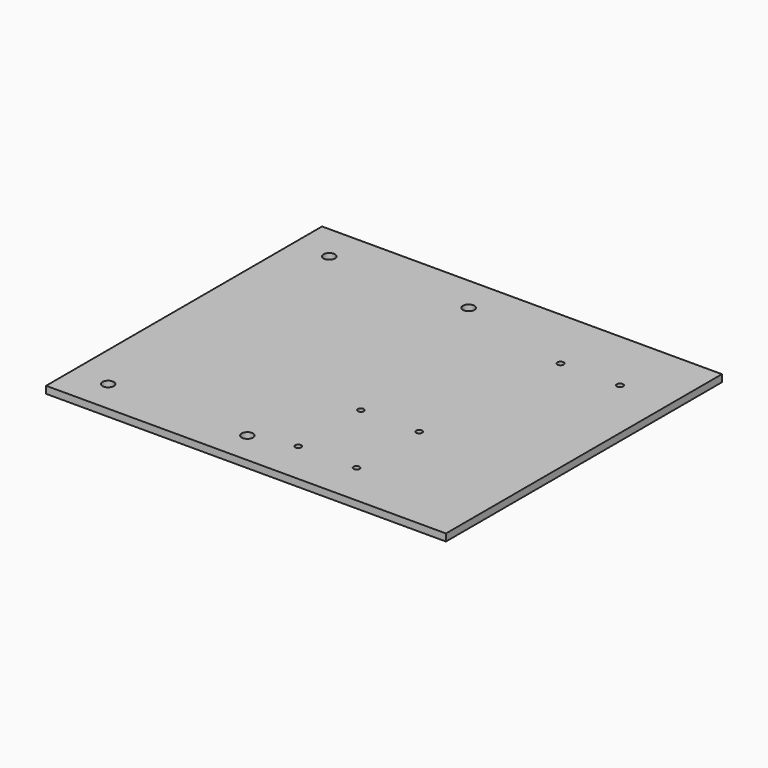
from build123d import *

# Parameters (mm, degrees)
F0_W     = 26
F0_H     = 35.5
F0_W_2   = 45
F0_H_2   = 10
F0_R     = 2
F0_R_2   = 1.05
F0_W_3   = 15
F0_R_3   = 1.1
F1_DEPTH = 2.5


with BuildPart() as f1:
    # F0 (on Top) → F1 (new body)
    with BuildSketch(Plane.XY):
        Polygon((-81.5970200658, 98.7071764616), (-96.5970200658, 98.7071764616), (-96.5970200658, -22.0728235384), (43.4029799342, -22.0728235384), (43.4029799342, 98.7071764616), (-36.5970200658, 98.7071764616), (-36.5970200658, 88.7071764616), (-35.1970200658, 88.7071764616), (-32.5970200658, 88.7071764616), (-32.5970200658, 86.1071764616), (-32.5970200658, -10.6928235384), (-32.5970200658, -13.2928235384), (-35.1970200658, -13.2928235384), (-83.9970200658, -13.2928235384), (-86.5970200658, -13.2928235384), (-86.5970200658, -10.6928235384), (-86.5970200658, 86.1071764616), (-86.5970200658, 86.5071764616), (-86.5970200658, 88.7071764616), (-84.3970200658, 88.7071764616), (-83.9970200658, 88.7071764616), (-81.5970200658, 88.7071764616), align=None)
        Polygon((-23.1610157355, -9.7928235384), (-23.1610157355, 23.2071764616), (-17.1610157355, 23.2071764616), (-17.1610157355, 33.2071764616), (-2.1610157355, 33.2071764616), (-2.1610157355, 23.2071764616), (2.8389842645, 23.2071764616), (2.8389842645, -9.7928235384), align=None, mode=Mode.SUBTRACT)
        with Locations((15.4029799342, 60.9571764616)):
            Rectangle(F0_W, F0_H, mode=Mode.SUBTRACT)
        with Locations((-59.0970200658, 93.7071764616)):
            Rectangle(F0_W_2, F0_H_2)
        Polygon((-36.5970200658, 88.7071764616), (-81.5970200658, 88.7071764616), (-83.9970200658, 88.7071764616), (-84.3970200658, 88.7071764616), (-86.5970200658, 88.7071764616), (-86.5970200658, 86.5071764616), (-86.5970200658, 86.1071764616), (-86.5970200658, -10.6928235384), (-86.5970200658, -13.2928235384), (-83.9970200658, -13.2928235384), (-35.1970200658, -13.2928235384), (-32.5970200658, -13.2928235384), (-32.5970200658, -10.6928235384), (-32.5970200658, 86.1071764616), (-32.5970200658, 88.7071764616), (-35.1970200658, 88.7071764616), align=None)
        with Locations((-83.9970200658, -10.6928235384)):
            Circle(F0_R, mode=Mode.SUBTRACT)
        with Locations((-35.1970200658, -10.6928235384)):
            Circle(F0_R, mode=Mode.SUBTRACT)
        with Locations((-83.9970200658, 86.1071764616)):
            Circle(F0_R, mode=Mode.SUBTRACT)
        with Locations((-35.1970200658, 86.1071764616)):
            Circle(F0_R, mode=Mode.SUBTRACT)
        Polygon((-17.1610157355, 23.2071764616), (-23.1610157355, 23.2071764616), (-23.1610157355, -9.7928235384), (2.8389842645, -9.7928235384), (2.8389842645, 23.2071764616), (-2.1610157355, 23.2071764616), align=None)
        with Locations((-20.3610157355, -6.9928235384)):
            Circle(F0_R_2, mode=Mode.SUBTRACT)
        with Locations((0.0389842645, -6.9928235384)):
            Circle(F0_R_2, mode=Mode.SUBTRACT)
        with Locations((-20.3610157355, 20.4071764616)):
            Circle(F0_R_2, mode=Mode.SUBTRACT)
        with Locations((0.0389842645, 20.4071764616)):
            Circle(F0_R_2, mode=Mode.SUBTRACT)
        with Locations((-9.6610157355, 28.2071764616)):
            Rectangle(F0_W_3, F0_H_2)
        with Locations((15.4029799342, 60.9571764616)):
            Rectangle(F0_W, F0_H)
        with Locations((5.0029799342, 76.1071764616)):
            Circle(F0_R_3, mode=Mode.SUBTRACT)
        with Locations((25.8029799342, 76.1071764616)):
            Circle(F0_R_3, mode=Mode.SUBTRACT)
    extrude(amount=F1_DEPTH)


solid = f1.part
